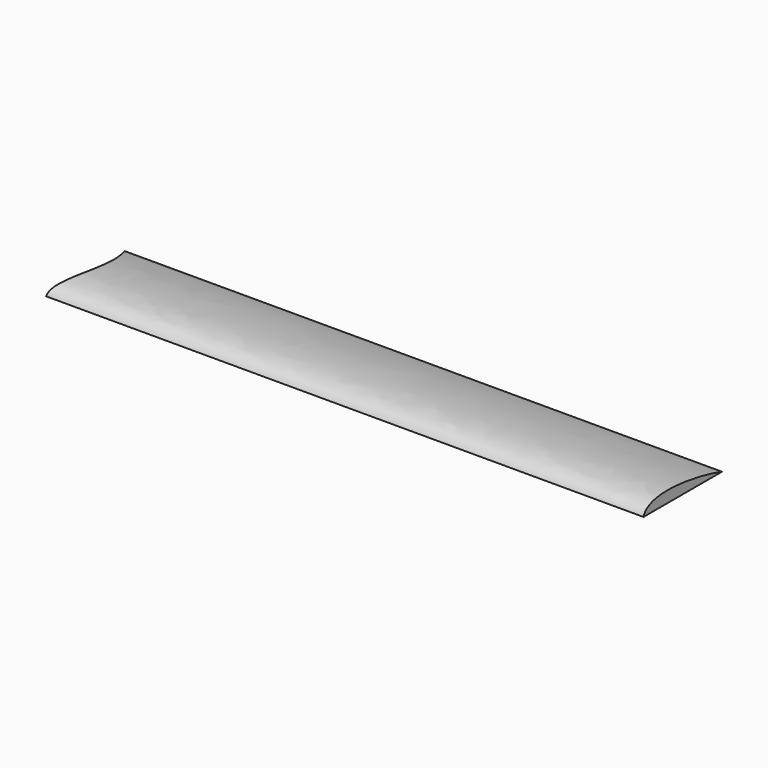
from build123d import *

# Parameters (mm, degrees)
F1_DEPTH = 39.116
F3_DEPTH = 7.62


with BuildPart() as f1:
    # F0 (on Right) → F1 (new body)
    with BuildSketch(Plane.YZ):
        with BuildLine():
            Line((-3.9117249368, 0), (2.4382750632, 0))
            add(Edge.make_bspline(
                [(-3.9117249368, 0), (-3.4905097758, 1.3348967768), (0.7074167952, 0.5567445187), (2.4382750632, 0)],
                knots=[0, 0, 0, 0, 6.35, 6.35, 6.35, 6.35], degree=3))
        make_face()
    extrude(amount=F1_DEPTH)

    # F2 (on face) → F3 (cut)
    with BuildSketch(Plane(origin=(0, 0, 0), x_dir=(1, 0, 0), z_dir=(0, 0, -1))):
        with BuildLine():
            ThreePointArc((0.419261314, -2.4382750632), (1.0536289969, -0.9067759996), (1.27, 0.7367249368))
            ThreePointArc((1.27, 0.7367249368), (1.0536289969, 2.3802258732), (0.419261314, 3.9117249368))
            Line((0.419261314, 3.9117249368), (0, 3.9117249368))
            Line((0, 3.9117249368), (0, 0.7367249368))
            Line((0, 0.7367249368), (0, -2.4382750632))
            Line((0, -2.4382750632), (0.419261314, -2.4382750632))
        make_face()
    extrude(amount=-F3_DEPTH, mode=Mode.SUBTRACT)


solid = f1.part
